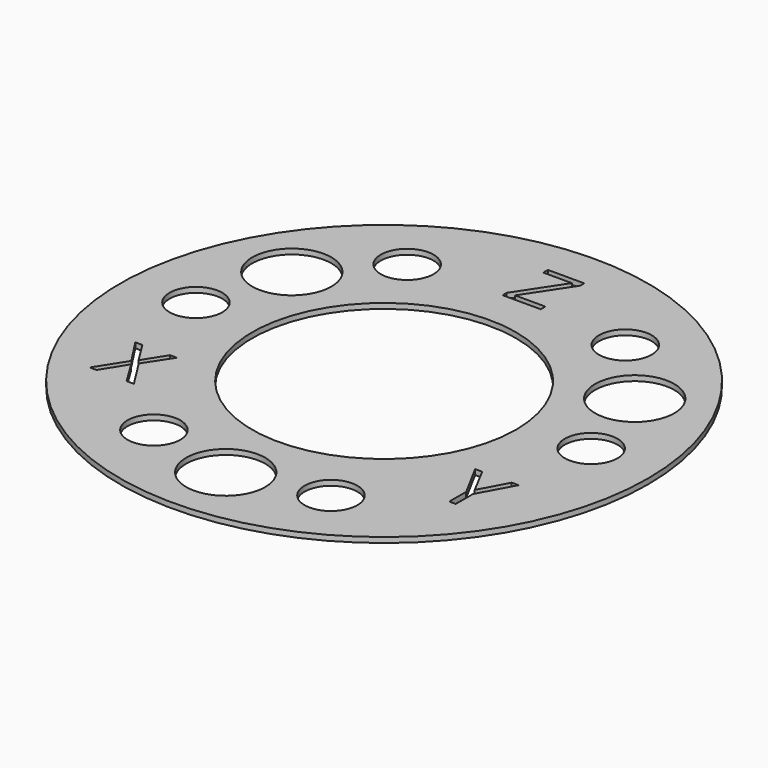
from build123d import *

# Parameters (mm, degrees)
F0_R         = 50
F0_R_2       = 25
F1_DEPTH     = 1
F2_R         = 7.5
F2_R_2       = 5
F2_TEXT_SIZE = 14.7246380544
F3_DEPTH     = 1.001


# Not quite as in the source:
# - Text() gives the source's letters only with a copy of the font that has no kerning and outlines rounded to 1/6400 em; it was checked with that copy


with BuildPart() as f1:
    # F0 (on Top) → F1 (new body)
    with BuildSketch(Plane.XY):
        Circle(F0_R)
        Circle(F0_R_2, mode=Mode.SUBTRACT)
    extrude(amount=F1_DEPTH)

    # F2 (on face) → F3 (cut, through all)
    with BuildSketch(Plane.XY.offset(1)):
        with Locations((-32.4759526419, 18.75)):
            Circle(F2_R)
        with Locations((-20.6607098961, 31.2951284801)):
            Circle(F2_R_2)
        with Locations((-37.4327312266, 2.2451353902)):
            Circle(F2_R_2)
        with Locations((37.4327312266, 2.2451353902)):
            Circle(F2_R_2)
        with Locations((32.4759526419, 18.75)):
            Circle(F2_R)
        with Locations((20.6607098961, 31.2951284801)):
            Circle(F2_R_2)
        with Locations((16.7720213304, -33.5402638703)):
            Circle(F2_R_2)
        with Locations((0, -37.5)):
            Circle(F2_R)
        with Locations((-16.7720213304, -33.5402638703)):
            Circle(F2_R_2)
        with Locations((-36.768052727, -23.8318517804)):
            Text('X', F2_TEXT_SIZE, font='Open Sans', text_align=(TextAlign.LEFT, TextAlign.BOTTOM))
        with Locations((28.1557347625, -24.1410909221)):
            Text('Y', F2_TEXT_SIZE, font='Open Sans', text_align=(TextAlign.LEFT, TextAlign.BOTTOM))
        with Locations((-4.0697776712, 32.4094779789)):
            Text('Z', F2_TEXT_SIZE, font='Open Sans', text_align=(TextAlign.LEFT, TextAlign.BOTTOM))
    extrude(amount=-F3_DEPTH, mode=Mode.SUBTRACT)


solid = f1.part
